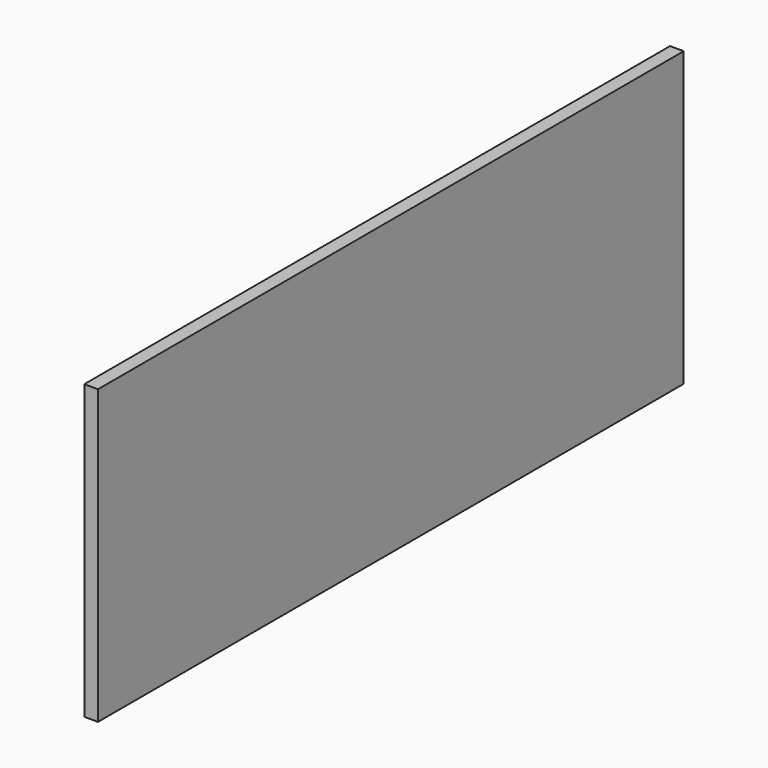
from build123d import *

# Parameters (mm, degrees)
F0_W     = 254
F0_H     = 101.6
F1_DEPTH = 4.7625


# Not quite as in the source:
# - a length typed as a fraction of an inch, garbled in the dataset ("3 / 203.2 mm" for 3/8 in), is restored


with BuildPart() as f1:
    # F0 (on Right) → F1 (new body)
    with BuildSketch(Plane.YZ):
        with Locations((17.0268568486, 12.6747479189)):
            Rectangle(F0_W, F0_H)
    extrude(amount=F1_DEPTH)


solid = f1.part
